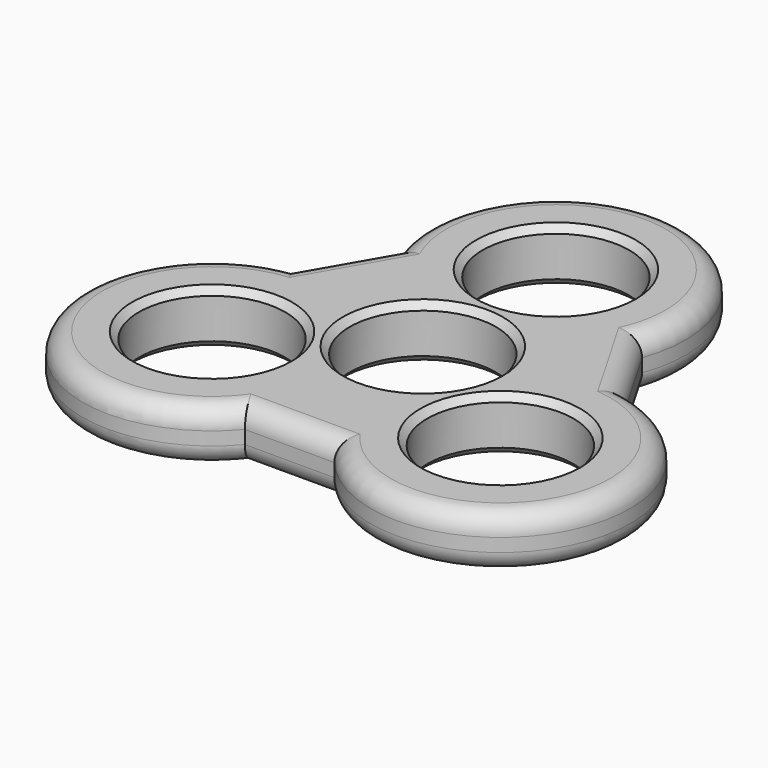
from build123d import *

# Parameters (mm, degrees)
F0_R      = 11
F1_DEPTH  = 4
F2_R      = 3
F3_SIZE   = 1
F4_SIZE   = 1
F7_R      = 2
F9_W      = 18.3584671468
F9_H      = 18.2486437261
F10_DEPTH = 25


with BuildPart() as f1:
    # F0 (on Top) → F1 (new body, symmetric)
    with BuildSketch(Plane.XY):
        with BuildLine():
            Line((25.0075728432, 6.6856132616), (18.293697346, 18.3143867384))
            ThreePointArc((18.293697346, 18.3143867384), (0, 44.4770836439), (-18.293697346, 18.3143867384))
            Line((-18.293697346, 18.3143867384), (-25.0075728432, 6.6856132616))
            ThreePointArc((-25.0075728432, 6.6856132616), (-38.5182843218, -22.2385418219), (-6.7138754972, -25))
            Line((-6.7138754972, -25), (6.7138754972, -25))
            ThreePointArc((6.7138754972, -25), (38.5182843218, -22.2385418219), (25.0075728432, 6.6856132616))
        make_face()
        with Locations((-21.6506350946, -12.5)):
            Circle(F0_R, mode=Mode.SUBTRACT)
        Circle(F0_R, mode=Mode.SUBTRACT)
        with Locations((21.6506350946, -12.5)):
            Circle(F0_R, mode=Mode.SUBTRACT)
        with Locations((0, 25)):
            Circle(F0_R, mode=Mode.SUBTRACT)
    extrude(amount=F1_DEPTH, both=True)

    # F2
    f2_edges = [f1.edges().sort_by_distance(p)[0] for p in [
        (38.518284, -22.238542, 4),
        (21.650635, 12.5, 4),
        (0, 44.477084, 4),
        (-21.650635, 12.5, 4),
        (-38.518284, -22.238542, 4),
        (0, -25, 4),
        (0, 44.477084, -4),
        (-38.518284, -22.238542, -4),
        (0, -25, -4),
        (38.518284, -22.238542, -4),
        (21.650635, 12.5, -4),
        (-21.650635, 12.5, -4),
    ]]
    fillet(f2_edges, radius=F2_R)

    # F3
    f3_edges = [f1.edges().sort_by_distance(p)[0] for p in [
        (-11, 25, 4),
        (-11, 0, 4),
        (-32.650635, -12.5, 4),
        (10.650635, -12.5, 4),
    ]]
    chamfer(f3_edges, length=F3_SIZE)

    # F4
    f4_edges = [f1.edges().sort_by_distance(p)[0] for p in [
        (-32.650635, -12.5, -4),
        (-11, 0, -4),
        (10.650635, -12.5, -4),
        (-11, 25, -4),
    ]]
    chamfer(f4_edges, length=F4_SIZE)


with BuildPart() as f6:
    # F5 (on Front) → F6 (revolve)
    with BuildSketch(Plane.XZ):
        with BuildLine():
            Line((0, 14.2753121717), (-28, 14.2753121717))
            ThreePointArc((-28, 14.2753121717), (-18.4101931298, 12.0795932054), (-10.7311751725, 5.9299378656))
            Line((-10.7311751725, 5.9299378656), (-9, -3.4046054352))
            Line((-9, -3.4046054352), (0, -3.4046054352))
            Line((0, -3.4046054352), (0, 0))
            Line((0, 0), (0, 14.2753121717))
        make_face()
    revolve(axis=Axis((0, 0, 7.1376560859), (0, 0, -1)))

    # F7#2 (call 1 of 2: OpenCascade refuses the feature's edges together)
    f7_2_edges = [f6.edges().sort_by_distance(p)[0] for p in [
        (9, 0, -3.404605),
    ]]
    fillet(f7_2_edges, radius=F7_R)

    # F7 (call 2 of 2)
    f7_edges = [f6.edges().sort_by_distance(p)[0] for p in [
        (28, 0, 14.275312),
    ]]
    fillet(f7_edges, radius=F7_R)


with BuildPart() as f10:
    # F9 (on Top) → F10 (new body)
    with BuildSketch(Plane.XY):
        with Locations((-28.5149300471, -59.2835787684)):
            Rectangle(F9_W, F9_H)
    extrude(amount=F10_DEPTH)


solid = f1.part
